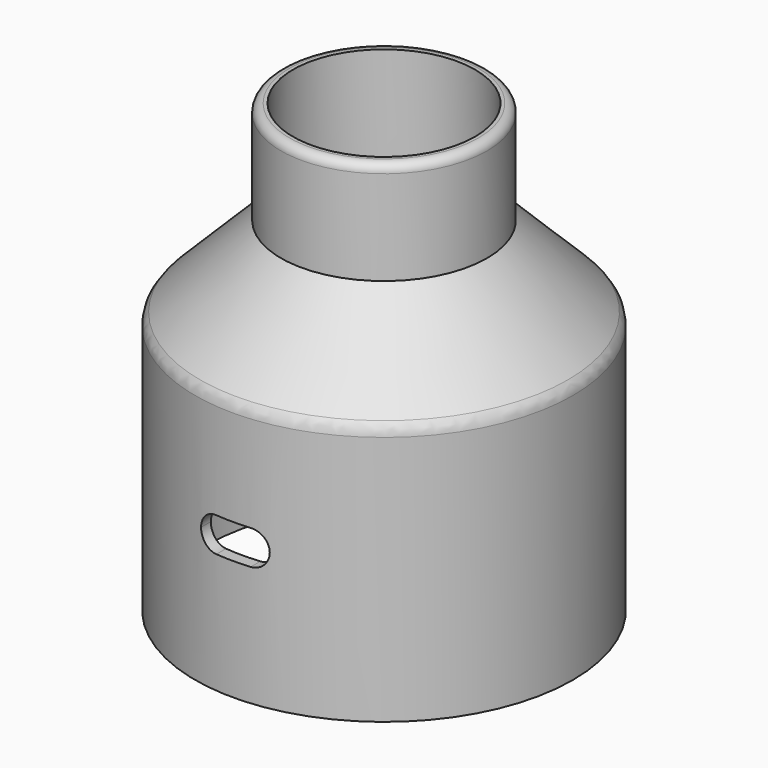
from build123d import *

# Parameters (mm, degrees)
F0_R     = 11
F1_DEPTH = 20
F2_SIZE  = 5
F3_DEPTH = 6
F4_T     = -0.7
F5_W     = 4
F5_H     = 2
F6_DEPTH = 12.5
F7_R     = 0.99999
F8_R     = 0.5
F9_R     = 1


# Not quite as in the source:
# - a fillet or chamfer is up to 0.001 mm smaller than in the source, because OpenCascade refuses the exact size


with BuildPart() as f1:
    # F0 (on Top) → F1 (new body)
    with BuildSketch(Plane.XY):
        Circle(F0_R)
    extrude(amount=F1_DEPTH)

    # F2
    f2_edges = [f1.edges().sort_by_distance(p)[0] for p in [
        (-11, 0, 20),
    ]]
    chamfer(f2_edges, length=F2_SIZE)

    # F3 (add): a face of the model
    f3_faces = [f1.faces().sort_by_distance(p)[0] for p in [
        (0, 0, 20),
    ]]
    extrude(f3_faces, amount=F3_DEPTH)

    # F4
    f4_openings = [f1.faces().sort_by_distance(p)[0] for p in [
        (0, 0, 26),
        (0, 0, 0),
    ]]
    offset(amount=F4_T, openings=f4_openings, kind=Kind.INTERSECTION)

    # F5 (on Front) → F6 (cut, symmetric)
    with BuildSketch(Plane.XZ):
        with Locations((0, 8)):
            Rectangle(F5_W, F5_H)
    extrude(amount=F6_DEPTH, both=True, mode=Mode.SUBTRACT)

    # F7 (radius 1 in the source; OpenCascade refuses exactly that, so slightly less here)
    f7_edges = [f1.edges().sort_by_distance(p)[0] for p in [
        (-2, 10.460307, 7),
        (-2, -10.460307, 7),
        (2, 10.460307, 9),
        (2, -10.460307, 9),
        (-2, 10.460307, 9),
        (-2, -10.460307, 9),
        (2, 10.460307, 7),
        (2, -10.460307, 7),
    ]]
    fillet(f7_edges, radius=F7_R)

    # F8
    f8_edges = [f1.edges().sort_by_distance(p)[0] for p in [
        (-6, 0, 26),
    ]]
    fillet(f8_edges, radius=F8_R)

    # F9
    f9_edges = [f1.edges().sort_by_distance(p)[0] for p in [
        (-11, 0, 15),
    ]]
    fillet(f9_edges, radius=F9_R)


solid = f1.part
